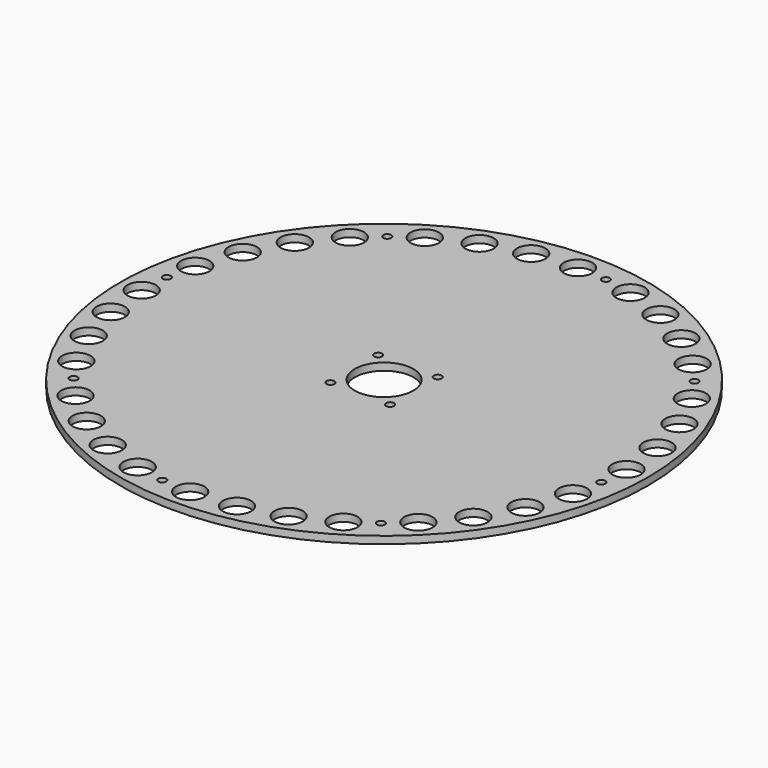
from build123d import *

# Parameters (mm, degrees)
F0_R            = 114.3
F0_R_2          = 1.7272
F0_R_3          = 12.7
F1_DEPTH        = 3.175
F2_R            = 6.1483621
F2_R_2          = 1.7272
F3_DEPTH        = 3.175
F3_COPIES_COUNT = 8


# Not quite as in the source:
# - a pattern or mirror of a feature is missing from the dataset's text; its kind, count and spacing are read off the source's solid


with BuildPart() as f1:
    # F0 (on Top) → F1 (new body)
    with BuildSketch(Plane.XY):
        Circle(F0_R)
        with Locations((-12.909118174, -12.909118174)):
            Circle(F0_R_2, mode=Mode.SUBTRACT)
        with Locations((12.909118174, -12.909118174)):
            Circle(F0_R_2, mode=Mode.SUBTRACT)
        with Locations((-12.909118174, 12.909118174)):
            Circle(F0_R_2, mode=Mode.SUBTRACT)
        Circle(F0_R_3, mode=Mode.SUBTRACT)
        with Locations((12.909118174, 12.909118174)):
            Circle(F0_R_2, mode=Mode.SUBTRACT)
    extrude(amount=F1_DEPTH)

    # F2 (on face) → F3 (cut, through all)
    with BuildSketch(Plane.XY.offset(3.175)):
        with Locations((-104.9766379, 0)):
            Circle(F2_R)
        with Locations((-103.2599191691, -18.9072366561)):
            Circle(F2_R)
        with Locations((-98.1659111494, -37.1960803446)):
            Circle(F2_R)
        with Locations((-89.8612219386, -54.2683636799)):
            Circle(F2_R)
        with Locations((-104.2084193553, 12.676744072)):
            Circle(F2_R_2)
    f3 = extrude(amount=-F3_DEPTH, mode=Mode.SUBTRACT)

    # F3_copies: F3 ×8 about axis
    f3_copies_axis = Axis((0, 0, 0), (0, 0, 1))
    for i in range(1, F3_COPIES_COUNT):
        add(f3.rotate(f3_copies_axis, i * 360 / F3_COPIES_COUNT), mode=Mode.SUBTRACT)


solid = f1.part
